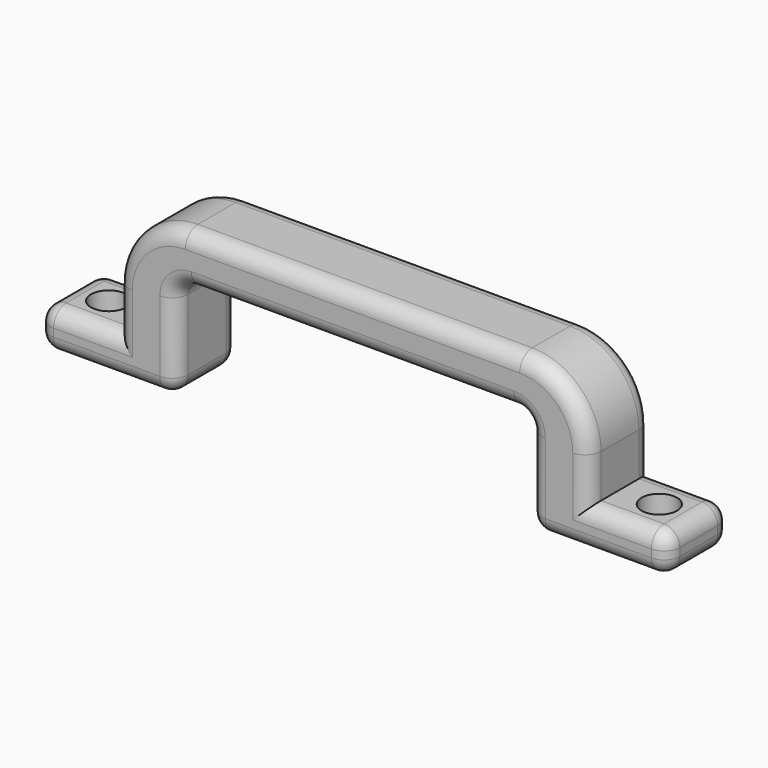
from build123d import *

# Parameters (mm, degrees)
F0_W         = 40
F0_H         = 20
F1_DEPTH     = 40
F2_R         = 9
F3_DEPTH     = 74.7
F4_R         = 8
F5_T1_DEPTH  = 40
F5_T4_ANGLE  = 90
F5_T6_ANGLE  = 90
F5_T8_ANGLE  = 90
F5_T10_ANGLE = 90


# Not quite as in the source:
# - a fillet or chamfer that OpenCascade refuses, or shapes differently, is made with other operations: its cross-section is extruded or revolved along the edge and cut away or added
# - a pattern or mirror of a feature is missing from the dataset's text; its kind, count and spacing are read off the source's solid


with BuildPart() as f1:
    # F0 (on Front) → F1 (new body)
    with BuildSketch(Plane.XZ):
        Polygon((-120, 20), (-120, 0), (-90, 0), (-90, 52), (0, 52), (90, 52), (90, 0), (120, 0), (160, 0), (160, 20), (120, 20), (120, 52), (120, 77), (0, 77), (-120, 77), (-120, 52), align=None)
        with Locations((-140, 10)):
            Rectangle(F0_W, F0_H)
    extrude(amount=F1_DEPTH)

    # F2 (on face) → F3 (cut)
    with BuildSketch(Plane.XY.offset(20)):
        with Locations((-140, -20)):
            Circle(F2_R)
    f3 = extrude(amount=-F3_DEPTH, mode=Mode.SUBTRACT)

    # F3_copies: F3 across plane
    add(f3.mirror(Plane(origin=(0, 0, 0), x_dir=(0, 0, 1), z_dir=(1, 0, 0))), mode=Mode.SUBTRACT)

    # F4
    f4_edges = [f1.edges().sort_by_distance(p)[0] for p in [
        (-160, -40, 10),
        (-160, 0, 10),
        (160, 0, 10),
        (160, -40, 10),
        (140, 0, 20),
        (120, 0, 48.5),
        (0, 0, 77),
        (-120, 0, 48.5),
        (-140, 0, 20),
        (-140, -40, 20),
        (-120, -40, 48.5),
        (0, -40, 77),
        (120, -40, 48.5),
        (140, -40, 20),
        (160, -20, 20),
        (160, -20, 0),
        (90, 0, 26),
        (0, 0, 52),
        (-90, 0, 26),
        (-125, 0, 0),
        (-160, -20, 0),
        (-125, -40, 0),
        (-90, -40, 26),
        (0, -40, 52),
        (90, -40, 26),
        (125, -40, 0),
        (90, -20, 0),
        (90, -20, 52),
        (-90, -20, 52),
        (-160, -20, 20),
        (125, 0, 0),
        (-90, -20, 0),
    ]]
    fillet(f4_edges, radius=F4_R)

    # F5: fillet of radius 35 on 2 edges, made by hand

    # F5_s2 → F5_t1 (cut)
    with BuildSketch(Plane.XZ):
        with BuildLine():
            ThreePointArc((-120, 42), (-109.7487373415, 66.7487373415), (-85, 77))
            Line((-85, 77), (-120, 77))
            Line((-120, 77), (-120, 42))
        make_face()
        with BuildLine():
            ThreePointArc((85, 77), (109.7487373415, 66.7487373415), (120, 42))
            Line((120, 42), (120, 77))
            Line((120, 77), (85, 77))
        make_face()
    extrude(amount=F5_T1_DEPTH, mode=Mode.SUBTRACT)

    # F5_s3 → F5_t4 (revolve, cut)
    with BuildSketch(Plane.YZ.offset(85)):
        with BuildLine():
            ThreePointArc((0, 69), (-2.3431457505, 74.6568542495), (-8, 77))
            Line((-8, 77), (0, 77))
            Line((0, 77), (0, 69))
        make_face()
    revolve(axis=Axis((85, 0, 42), (0, 1, 0)), revolution_arc=F5_T4_ANGLE, mode=Mode.SUBTRACT)

    # F5_s5 → F5_t6 (revolve, cut)
    with BuildSketch(Plane.XY.offset(42)):
        with BuildLine():
            ThreePointArc((112, -40), (117.6568542495, -37.6568542495), (120, -32))
            Line((120, -32), (120, -40))
            Line((120, -40), (112, -40))
        make_face()
    revolve(axis=Axis((85, -40, 42), (0, -1, 0)), revolution_arc=F5_T6_ANGLE, mode=Mode.SUBTRACT)

    # F5_s7 → F5_t8 (revolve, cut)
    with BuildSketch(Plane.XY.offset(42)):
        with BuildLine():
            ThreePointArc((-112, 0), (-117.6568542495, -2.3431457505), (-120, -8))
            Line((-120, -8), (-120, 0))
            Line((-120, 0), (-112, 0))
        make_face()
    revolve(axis=Axis((-85, 0, 42), (0, 1, 0)), revolution_arc=F5_T8_ANGLE, mode=Mode.SUBTRACT)

    # F5_s9 → F5_t10 (revolve, cut)
    with BuildSketch(Plane.YZ.offset(-85)):
        with BuildLine():
            ThreePointArc((-40, 69), (-37.6568542495, 74.6568542495), (-32, 77))
            Line((-32, 77), (-40, 77))
            Line((-40, 77), (-40, 69))
        make_face()
    revolve(axis=Axis((-85, -40, 42), (0, -1, 0)), revolution_arc=F5_T10_ANGLE, mode=Mode.SUBTRACT)


solid = f1.part
